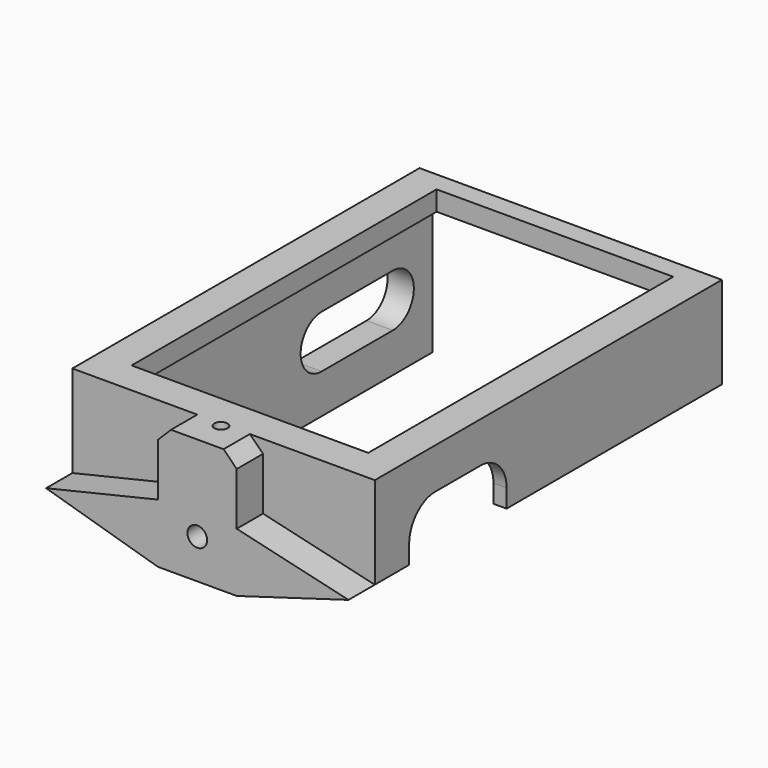
from build123d import *

# Parameters (mm, degrees)
F0_W          = 46
F0_H          = 66
F0_W_2        = 36
F0_H_2        = 58
F1_DEPTH      = 3
F2_W          = 2
F2_H          = 61
F2_H_2        = 5
F3_DEPTH      = 11
F5_DEPTH      = 2
F6_W          = 12
F6_H          = 10
F7_DEPTH      = 5
F7_DEPTH_BACK = 5
F8_R          = 1.5
F9_DEPTH      = 10
F10_R         = 1
F11_DEPTH     = 11.8829661115
F12_DEPTH     = 10
F14_DEPTH     = 2
F16_DEPTH     = 2
F17_R         = 5
F18_SIZE      = 2


with BuildPart() as f1:
    # F0 (on Top) → F1 (new body)
    with BuildSketch(Plane.XY):
        Rectangle(F0_W, F0_H)
        with Locations((0, 1)):
            Rectangle(F0_W_2, F0_H_2, mode=Mode.SUBTRACT)
    extrude(amount=F1_DEPTH)

    # F2 (on face) → F3 (join)
    with BuildSketch(Plane(origin=(0, 0, 0), x_dir=(1, 0, 0), z_dir=(0, 0, -1))):
        with Locations((-22, -2.5)):
            Rectangle(F2_W, F2_H)
        Polygon((18, 28), (21, 28), (21, 33), (-23, 33), (-23, 28), (-21, 28), (-18, 28), align=None)
        with Locations((22, -2.5)):
            Rectangle(F2_W, F2_H)
        with Locations((22, 30.5)):
            Rectangle(F2_W, F2_H_2)
    extrude(amount=F3_DEPTH)

    # F4 (on face) → F5 (cut, through all)
    with BuildSketch(Plane.YZ.offset(23)):
        with BuildLine():
            Line((-26.4700967818, -11), (-7.943155244, -11))
            Line((-7.943155244, -11), (-7.943155244, -8.2140678056))
            ThreePointArc((-7.943155244, -8.2140678056), (-9.4076213381, -4.6785338996), (-12.943155244, -3.2140678056))
            Line((-12.943155244, -3.2140678056), (-21.4700967818, -3.2140678056))
            ThreePointArc((-21.4700967818, -3.2140678056), (-25.0056306878, -4.6785338996), (-26.4700967818, -8.2140678056))
            Line((-26.4700967818, -8.2140678056), (-26.4700967818, -11))
        make_face()
    extrude(amount=-F5_DEPTH, mode=Mode.SUBTRACT)

    # F6 (on face) → F7 (join, two sides)
    with BuildSketch(Plane.XZ.offset(33)) as f7_sk:
        with Locations((0, -2)):
            Rectangle(F6_W, F6_H)
        Polygon((23, -11), (6, -7), (-6, -7), (-23, -11), (-6, -16), (6, -16), align=None)
    extrude(amount=F7_DEPTH)
    extrude(f7_sk.sketch, amount=-F7_DEPTH_BACK)

    # F8 (on face) → F9 (cut, through all)
    with BuildSketch(Plane.XZ.offset(38)):
        with Locations((0, -10)):
            Circle(F8_R)
    extrude(amount=-F9_DEPTH, mode=Mode.SUBTRACT)

    # F10 (on face) → F11 (cut, through all)
    with BuildSketch(Plane.XY.offset(3)):
        with Locations((0, -33.5)):
            Circle(F10_R)
    extrude(amount=-F11_DEPTH, mode=Mode.SUBTRACT)

    # F12 (add): a face of the model
    f12_faces = [f1.faces().sort_by_distance(p)[0] for p in [
        (-22, 2.5, -11),
    ]]
    extrude(f12_faces, amount=F12_DEPTH)

    # F13 (on face) → F14 (cut, through all)
    with BuildSketch(Plane(origin=(-23, 0, 0), x_dir=(0, -1, 0), z_dir=(-1, 0, 0))):
        with BuildLine():
            ThreePointArc((-25.4259229114, -7), (-29.4259229114, -11), (-25.4259229114, -15))
            Line((-25.4259229114, -15), (-11.899846606, -15))
            ThreePointArc((-11.899846606, -15), (-7.899846606, -11), (-11.899846606, -7))
            Line((-11.899846606, -7), (-25.4259229114, -7))
        make_face()
    extrude(amount=-F14_DEPTH, mode=Mode.SUBTRACT)

    # F15 (on face) → F16 (join)
    with BuildSketch(Plane(origin=(-23, 0, 0), x_dir=(0, -1, 0), z_dir=(-1, 0, 0))):
        with BuildLine():
            ThreePointArc((-25.4259229114, -4), (-32.4259229114, -11), (-25.4259229114, -18))
            Line((-25.4259229114, -18), (-11.899846606, -18))
            ThreePointArc((-11.899846606, -18), (-4.899846606, -11), (-11.899846606, -4))
            Line((-11.899846606, -4), (-25.4259229114, -4))
        make_face()
        with BuildLine():
            Line((-11.899846606, -15), (-25.4259229114, -15))
            ThreePointArc((-25.4259229114, -15), (-29.4259229114, -11), (-25.4259229114, -7))
            Line((-25.4259229114, -7), (-11.899846606, -7))
            ThreePointArc((-11.899846606, -7), (-7.899846606, -11), (-11.899846606, -15))
        make_face(mode=Mode.SUBTRACT)
    extrude(amount=F16_DEPTH)

    # F17
    f17_edges = [f1.edges().sort_by_distance(p)[0] for p in [
        (-22, -28, -21),
    ]]
    fillet(f17_edges, radius=F17_R)

    # F18
    f18_edges = [f1.edges().sort_by_distance(p)[0] for p in [
        (6, -35.5, 3),
        (-6, -35.5, 3),
    ]]
    chamfer(f18_edges, length=F18_SIZE)


solid = f1.part
